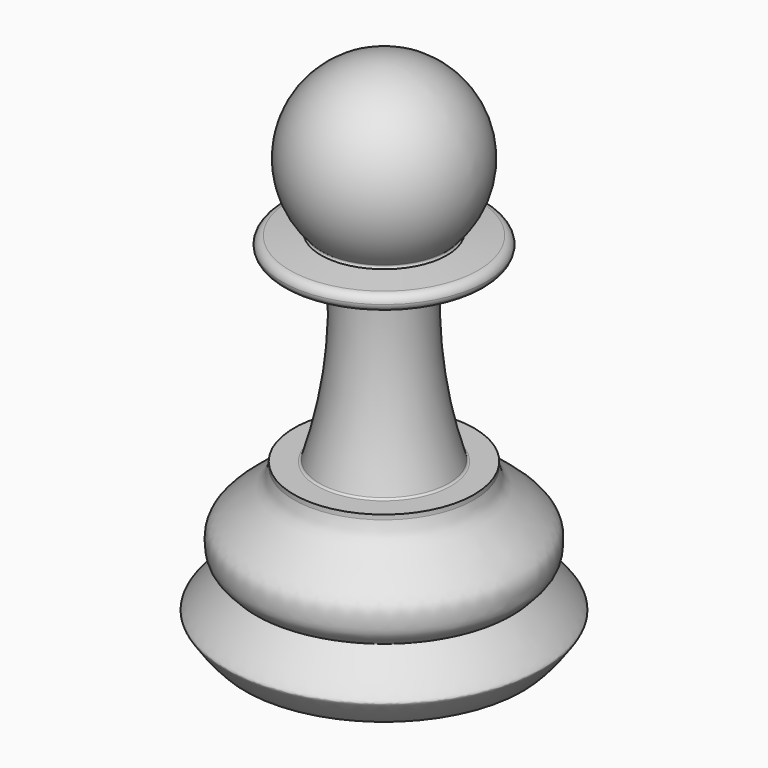
from build123d import *


with BuildPart() as f1:
    # F0 (on Front) → F1 (revolve)
    with BuildSketch(Plane.XZ):
        with BuildLine():
            Line((19, -57.3077059366), (0, -57.3077059366))
            Line((0, -57.3077059366), (0, -89.4568003867))
            Line((0, -89.4568003867), (29.3, -89.4568003867))
            add(Edge.make_bspline(
                [(26.9592367113, -76.1797651649), (29.5225490997, -78.9538033711), (33.0190249664, -82.727702405), (33.6161066802, -83.9052734845), (33.0561881237, -84.7180951511), (30.9753428321, -87.8290817836), (29.3, -89.4568003867)],
                knots=[0, 0, 0, 0, 0.4124161473, 0.5428121985, 0.6615346774, 1, 1, 1, 1], degree=3))
            add(Edge.make_bspline(
                [(19, -57.3077059366), (19.3947468179, -59.1347886267), (20.5064753127, -61.3937856627), (29.8925378169, -67.2108287114), (29.4876468568, -71.6376547275), (29.3237060979, -74.1535690433), (26.8095991963, -76.1395467772), (26.9592367113, -76.1797651649)],
                knots=[0, 0, 0, 0, 0.202479402, 0.5042329978, 0.6898433279, 0.8476886808, 1, 1, 1, 1], degree=3))
        make_face()
        with BuildLine():
            ThreePointArc((13.2853137329, -13.7159600853), (13.0558026627, -13.3893818497), (13.1587623714, -13.0037291903))
            ThreePointArc((13.1587623714, -13.0037291903), (17.070720401, 7.1302527999), (0, 18.5))
            Line((0, 18.5), (0, -57.3077059366))
            Line((0, -57.3077059366), (19, -57.3077059366))
            Line((19, -57.3077059366), (19, -56.3077059366))
            Line((19, -56.3077059366), (16.9227282165, -56.3077059366))
            Line((16.9227282165, -56.3077059366), (14.1160641541, -56.3077059366))
            ThreePointArc((14.1160641541, -56.3077059366), (13.8203106422, -56.2108558594), (13.6391321322, -55.9578253776))
            ThreePointArc((13.6391321322, -55.9578253776), (9.7976220598, -37.6566938703), (9.5953075204, -18.9578253776))
            Line((9.5953075204, -18.9578253776), (19.9387038202, -17.6779447283))
            ThreePointArc((19.9387038202, -17.6779447283), (21.0335140908, -17.1197896987), (21.5150116553, -15.9891674537))
            ThreePointArc((21.5150116553, -15.9891674537), (21.0007400429, -14.8774857988), (19.8941887936, -14.352266106))
            Line((19.8941887936, -14.352266106), (13.2853137329, -13.7159600853))
        make_face()
    revolve(axis=Axis((0, 0, -1.5011268521), (0, 0, -1)))


solid = f1.part
